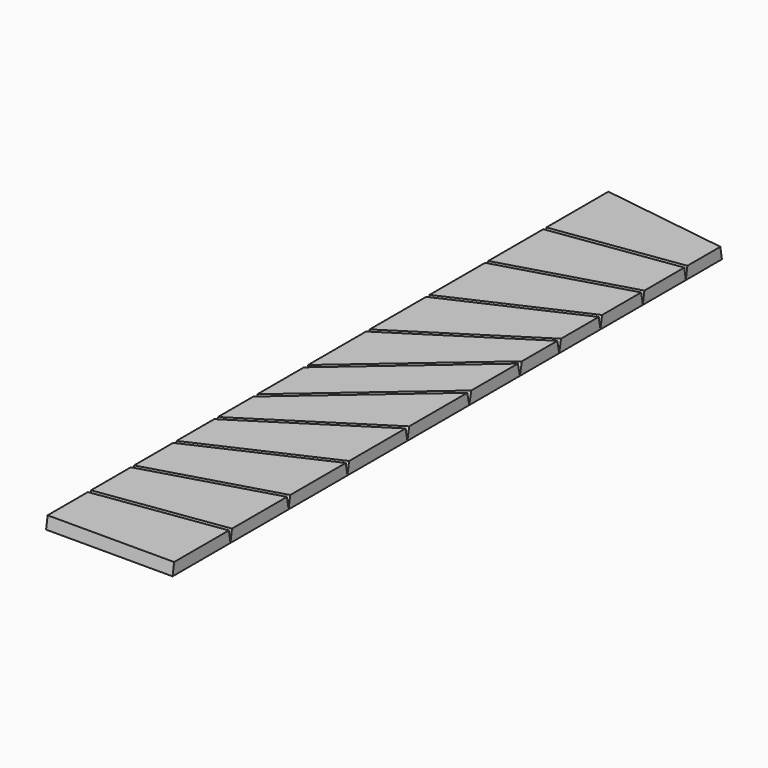
from build123d import *

# Parameters (mm, degrees)
F2_DEPTH    = 9.525
F3_DEPTH    = 9.525
F4_DEPTH    = 9.525
F5_DEPTH    = 9.525
F6_DEPTH    = 9.525
F7_DEPTH    = 9.525
F8_DEPTH    = 9.525
F9_DEPTH    = 9.525
F10_DEPTH   = 9.525
F11_DEPTH   = 9.525
F12_DEPTH   = 9.525
F13_SIZE2   = 1.550911
F13_SIZE    = 9.52499
F13_2_SIZE2 = 1.550911
F13_2_SIZE  = 9.52499
F14_SIZE2   = 1.550911
F14_SIZE    = 9.52499
F14_2_SIZE2 = 1.550911
F14_2_SIZE  = 9.52499
F15_SIZE2   = 1.550911
F15_SIZE    = 9.52499
F15_2_SIZE2 = 1.550911
F15_2_SIZE  = 9.52499
F16_SIZE2   = 1.550911
F16_SIZE    = 9.52499
F16_2_SIZE2 = 1.550911
F16_2_SIZE  = 9.52499
F17_SIZE2   = 1.550911
F17_SIZE    = 9.52499
F17_2_SIZE2 = 1.550911
F17_2_SIZE  = 9.52499
F18_SIZE2   = 1.550911
F18_SIZE    = 9.52499
F18_2_SIZE2 = 1.550911
F18_2_SIZE  = 9.52499
F19_SIZE2   = 1.550911
F19_SIZE    = 9.52499
F19_2_SIZE2 = 1.550911
F19_2_SIZE  = 9.52499
F20_SIZE2   = 1.550911
F20_SIZE    = 9.52499
F20_2_SIZE2 = 1.550911
F20_2_SIZE  = 9.52499
F21_SIZE2   = 1.550911
F21_SIZE    = 9.52499
F21_2_SIZE2 = 1.550911
F21_2_SIZE  = 9.52499
F22_SIZE2   = 1.550911
F22_SIZE    = 9.52499
F22_2_SIZE2 = 1.550911
F22_2_SIZE  = 9.52499
F23_SIZE2   = 1.550911
F23_SIZE    = 9.52499
F23_2_SIZE2 = 1.550911
F23_2_SIZE  = 9.52499


# Not quite as in the source:
# - a fillet or chamfer is up to 0.001 mm smaller than in the source, because OpenCascade refuses the exact size


with BuildPart() as f2:
    # F1 (on Top) → F2 (new body)
    with BuildSketch(Plane.XY):
        Polygon((-50.8, 279.4), (-50.8, 221.3135439188), (50.8, 235.8864560812), (50.8, 272.1135439188), (-50.8, 286.6864560812), align=None)
    extrude(amount=F2_DEPTH)

    # F13 (size 9.525 and 1.5509205186 in the source; OpenCascade refuses exactly that, so slightly less here)
    f13_edges = [f2.edges().sort_by_distance(p)[0] for p in [
        (0, 228.6, 9.525),
    ]]
    f13_side = f2.faces().sort_by_distance((0, 228.6, 4.7625))[0]
    chamfer(f13_edges, length=F13_SIZE, length2=F13_SIZE2, reference=f13_side)

    # F13#2 (size 9.525 and 1.5509205186 in the source; OpenCascade refuses exactly that, so slightly less here)
    f13_2_edges = [f2.edges().sort_by_distance(p)[0] for p in [
        (0, 279.4, 9.525),
    ]]
    f13_2_side = f2.faces().sort_by_distance((0, 279.4, 4.7625))[0]
    chamfer(f13_2_edges, length=F13_2_SIZE, length2=F13_2_SIZE2, reference=f13_2_side)


with BuildPart() as f3:
    # F1 (on Top) → F3 (new body)
    with BuildSketch(Plane.XY):
        Polygon((-50.8, 221.3135439188), (-50.8, 162.9209762891), (50.8, 192.6790237109), (50.8, 235.8864560812), align=None)
    extrude(amount=F3_DEPTH)

    # F14 (size 9.525 and 1.5509205186 in the source; OpenCascade refuses exactly that, so slightly less here)
    f14_edges = [f3.edges().sort_by_distance(p)[0] for p in [
        (0, 228.6, 9.525),
    ]]
    f14_side = f3.faces().sort_by_distance((0, 228.6, 4.7625))[0]
    chamfer(f14_edges, length=F14_SIZE, length2=F14_SIZE2, reference=f14_side)

    # F14#2 (size 9.525 and 1.5509205186 in the source; OpenCascade refuses exactly that, so slightly less here)
    f14_2_edges = [f3.edges().sort_by_distance(p)[0] for p in [
        (0, 177.8, 9.525),
    ]]
    f14_2_side = f3.faces().sort_by_distance((0, 177.8, 4.7625))[0]
    chamfer(f14_2_edges, length=F14_2_SIZE, length2=F14_2_SIZE2, reference=f14_2_side)


with BuildPart() as f4:
    # F1 (on Top) → F4 (new body)
    with BuildSketch(Plane.XY):
        Polygon((-50.8, 162.9209762891), (-50.8, 103.8624894848), (50.8, 150.1375105152), (50.8, 192.6790237109), align=None)
    extrude(amount=F4_DEPTH)

    # F15 (size 9.525 and 1.5509205186 in the source; OpenCascade refuses exactly that, so slightly less here)
    f15_edges = [f4.edges().sort_by_distance(p)[0] for p in [
        (0, 177.8, 9.525),
    ]]
    f15_side = f4.faces().sort_by_distance((0, 177.8, 4.7625))[0]
    chamfer(f15_edges, length=F15_SIZE, length2=F15_SIZE2, reference=f15_side)

    # F15#2 (size 9.525 and 1.5509205186 in the source; OpenCascade refuses exactly that, so slightly less here)
    f15_2_edges = [f4.edges().sort_by_distance(p)[0] for p in [
        (0, 127, 9.525),
    ]]
    f15_2_side = f4.faces().sort_by_distance((0, 127, 4.7625))[0]
    chamfer(f15_2_edges, length=F15_2_SIZE, length2=F15_2_SIZE2, reference=f15_2_side)


with BuildPart() as f5:
    # F1 (on Top) → F5 (new body)
    with BuildSketch(Plane.XY):
        Polygon((-50.8, 103.8624894848), (-50.8, 43.64954709), (50.8, 108.75045291), (50.8, 150.1375105152), align=None)
    extrude(amount=F5_DEPTH)

    # F16 (size 9.525 and 1.5509205186 in the source; OpenCascade refuses exactly that, so slightly less here)
    f16_edges = [f5.edges().sort_by_distance(p)[0] for p in [
        (0, 127, 9.525),
    ]]
    f16_side = f5.faces().sort_by_distance((0, 127, 4.7625))[0]
    chamfer(f16_edges, length=F16_SIZE, length2=F16_SIZE2, reference=f16_side)

    # F16#2 (size 9.525 and 1.5509205186 in the source; OpenCascade refuses exactly that, so slightly less here)
    f16_2_edges = [f5.edges().sort_by_distance(p)[0] for p in [
        (0, 76.2, 9.525),
    ]]
    f16_2_side = f5.faces().sort_by_distance((0, 76.2, 4.7625))[0]
    chamfer(f16_2_edges, length=F16_2_SIZE, length2=F16_2_SIZE2, reference=f16_2_side)


with BuildPart() as f6:
    # F1 (on Top) → F6 (new body)
    with BuildSketch(Plane.XY):
        Polygon((-50.8, 43.64954709), (-50.8, -18.4687277608), (50.8, 69.2687277608), (50.8, 108.75045291), align=None)
    extrude(amount=F6_DEPTH)

    # F17 (size 9.525 and 1.5509205186 in the source; OpenCascade refuses exactly that, so slightly less here)
    f17_edges = [f6.edges().sort_by_distance(p)[0] for p in [
        (0, 25.4, 9.525),
    ]]
    f17_side = f6.faces().sort_by_distance((0, 25.4, 4.7625))[0]
    chamfer(f17_edges, length=F17_SIZE, length2=F17_SIZE2, reference=f17_side)

    # F17#2 (size 9.525 and 1.5509205186 in the source; OpenCascade refuses exactly that, so slightly less here)
    f17_2_edges = [f6.edges().sort_by_distance(p)[0] for p in [
        (0, 76.2, 9.525),
    ]]
    f17_2_side = f6.faces().sort_by_distance((0, 76.2, 4.7625))[0]
    chamfer(f17_2_edges, length=F17_2_SIZE, length2=F17_2_SIZE2, reference=f17_2_side)


with BuildPart() as f7:
    # F1 (on Top) → F7 (new body)
    with BuildSketch(Plane.XY):
        Polygon((-50.8, -18.4687277608), (-50.8, -69.2687277608), (50.8, 18.4687277608), (50.8, 69.2687277608), align=None)
    extrude(amount=F7_DEPTH)

    # F18 (size 9.525 and 1.5509205186 in the source; OpenCascade refuses exactly that, so slightly less here)
    f18_edges = [f7.edges().sort_by_distance(p)[0] for p in [
        (0, 25.4, 9.525),
    ]]
    f18_side = f7.faces().sort_by_distance((0, 25.4, 4.7625))[0]
    chamfer(f18_edges, length=F18_SIZE, length2=F18_SIZE2, reference=f18_side)

    # F18#2 (size 9.525 and 1.5509205186 in the source; OpenCascade refuses exactly that, so slightly less here)
    f18_2_edges = [f7.edges().sort_by_distance(p)[0] for p in [
        (0, -25.4, 9.525),
    ]]
    f18_2_side = f7.faces().sort_by_distance((0, -25.4, 4.7625))[0]
    chamfer(f18_2_edges, length=F18_2_SIZE, length2=F18_2_SIZE2, reference=f18_2_side)


with BuildPart() as f8:
    # F1 (on Top) → F8 (new body)
    with BuildSketch(Plane.XY):
        Polygon((-50.8, -69.2687277608), (-50.8, -108.75045291), (50.8, -43.64954709), (50.8, 18.4687277608), align=None)
    extrude(amount=F8_DEPTH)

    # F19 (size 9.525 and 1.5509205186 in the source; OpenCascade refuses exactly that, so slightly less here)
    f19_edges = [f8.edges().sort_by_distance(p)[0] for p in [
        (0, -25.4, 9.525),
    ]]
    f19_side = f8.faces().sort_by_distance((0, -25.4, 4.7625))[0]
    chamfer(f19_edges, length=F19_SIZE, length2=F19_SIZE2, reference=f19_side)

    # F19#2 (size 9.525 and 1.5509205186 in the source; OpenCascade refuses exactly that, so slightly less here)
    f19_2_edges = [f8.edges().sort_by_distance(p)[0] for p in [
        (0, -76.2, 9.525),
    ]]
    f19_2_side = f8.faces().sort_by_distance((0, -76.2, 4.7625))[0]
    chamfer(f19_2_edges, length=F19_2_SIZE, length2=F19_2_SIZE2, reference=f19_2_side)


with BuildPart() as f9:
    # F1 (on Top) → F9 (new body)
    with BuildSketch(Plane.XY):
        Polygon((-50.8, -108.75045291), (-50.8, -150.1375105152), (50.8, -103.8624894848), (50.8, -43.64954709), align=None)
    extrude(amount=F9_DEPTH)

    # F20 (size 9.525 and 1.5509205186 in the source; OpenCascade refuses exactly that, so slightly less here)
    f20_edges = [f9.edges().sort_by_distance(p)[0] for p in [
        (0, -76.2, 9.525),
    ]]
    f20_side = f9.faces().sort_by_distance((0, -76.2, 4.7625))[0]
    chamfer(f20_edges, length=F20_SIZE, length2=F20_SIZE2, reference=f20_side)

    # F20#2 (size 9.525 and 1.5509205186 in the source; OpenCascade refuses exactly that, so slightly less here)
    f20_2_edges = [f9.edges().sort_by_distance(p)[0] for p in [
        (0, -127, 9.525),
    ]]
    f20_2_side = f9.faces().sort_by_distance((0, -127, 4.7625))[0]
    chamfer(f20_2_edges, length=F20_2_SIZE, length2=F20_2_SIZE2, reference=f20_2_side)


with BuildPart() as f10:
    # F1 (on Top) → F10 (new body)
    with BuildSketch(Plane.XY):
        Polygon((-50.8, -150.1375105152), (-50.8, -192.6790237109), (50.8, -162.9209762891), (50.8, -103.8624894848), align=None)
    extrude(amount=F10_DEPTH)

    # F21 (size 9.525 and 1.5509205186 in the source; OpenCascade refuses exactly that, so slightly less here)
    f21_edges = [f10.edges().sort_by_distance(p)[0] for p in [
        (0, -127, 9.525),
    ]]
    f21_side = f10.faces().sort_by_distance((0, -127, 4.7625))[0]
    chamfer(f21_edges, length=F21_SIZE, length2=F21_SIZE2, reference=f21_side)

    # F21#2 (size 9.525 and 1.5509205186 in the source; OpenCascade refuses exactly that, so slightly less here)
    f21_2_edges = [f10.edges().sort_by_distance(p)[0] for p in [
        (0, -177.8, 9.525),
    ]]
    f21_2_side = f10.faces().sort_by_distance((0, -177.8, 4.7625))[0]
    chamfer(f21_2_edges, length=F21_2_SIZE, length2=F21_2_SIZE2, reference=f21_2_side)


with BuildPart() as f11:
    # F1 (on Top) → F11 (new body)
    with BuildSketch(Plane.XY):
        Polygon((-50.8, -192.6790237109), (-50.8, -235.8864560812), (50.8, -221.3135439188), (50.8, -162.9209762891), align=None)
    extrude(amount=F11_DEPTH)

    # F22 (size 9.525 and 1.5509205186 in the source; OpenCascade refuses exactly that, so slightly less here)
    f22_edges = [f11.edges().sort_by_distance(p)[0] for p in [
        (0, -177.8, 9.525),
    ]]
    f22_side = f11.faces().sort_by_distance((0, -177.8, 4.7625))[0]
    chamfer(f22_edges, length=F22_SIZE, length2=F22_SIZE2, reference=f22_side)

    # F22#2 (size 9.525 and 1.5509205186 in the source; OpenCascade refuses exactly that, so slightly less here)
    f22_2_edges = [f11.edges().sort_by_distance(p)[0] for p in [
        (0, -228.6, 9.525),
    ]]
    f22_2_side = f11.faces().sort_by_distance((0, -228.6, 4.7625))[0]
    chamfer(f22_2_edges, length=F22_2_SIZE, length2=F22_2_SIZE2, reference=f22_2_side)


with BuildPart() as f12:
    # F1 (on Top) → F12 (new body)
    with BuildSketch(Plane.XY):
        Polygon((-50.8, -235.8864560812), (-50.8, -279.4), (50.8, -279.4), (50.8, -221.3135439188), align=None)
    extrude(amount=F12_DEPTH)

    # F23 (size 9.525 and 1.5509205186 in the source; OpenCascade refuses exactly that, so slightly less here)
    f23_edges = [f12.edges().sort_by_distance(p)[0] for p in [
        (0, -228.6, 9.525),
    ]]
    f23_side = f12.faces().sort_by_distance((0, -228.6, 4.7625))[0]
    chamfer(f23_edges, length=F23_SIZE, length2=F23_SIZE2, reference=f23_side)

    # F23#2 (size 9.525 and 1.5509205186 in the source; OpenCascade refuses exactly that, so slightly less here)
    f23_2_edges = [f12.edges().sort_by_distance(p)[0] for p in [
        (0, -279.4, 9.525),
    ]]
    f23_2_side = f12.faces().sort_by_distance((0, -279.4, 4.7625))[0]
    chamfer(f23_2_edges, length=F23_2_SIZE, length2=F23_2_SIZE2, reference=f23_2_side)


solid = Compound([f2.part, f3.part, f4.part, f5.part, f6.part, f7.part, f8.part, f9.part, f10.part, f11.part, f12.part])
